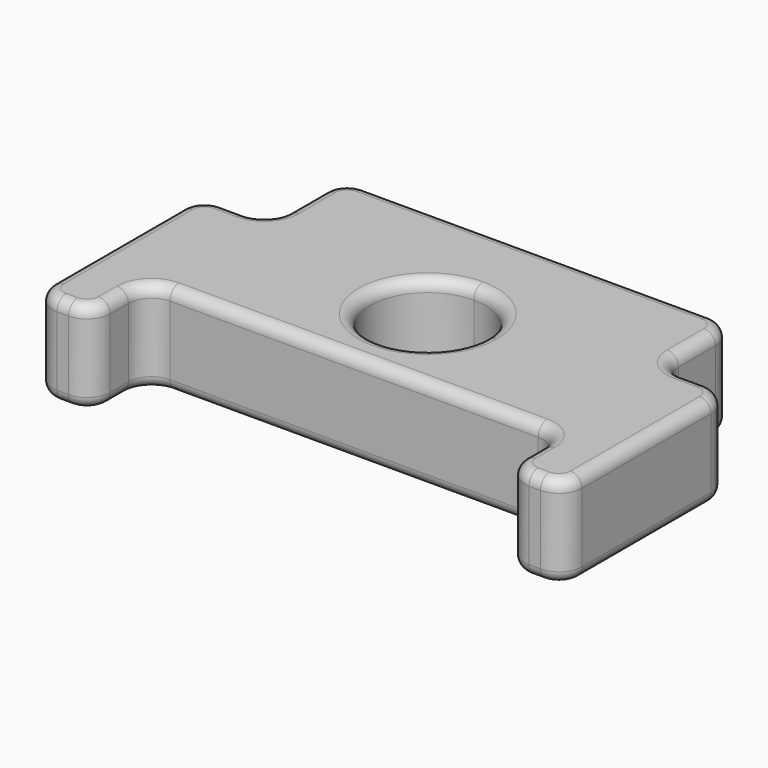
from build123d import *

# Parameters (mm, degrees)
F1_DEPTH = 4
F2_R     = 1
F3_R     = 0.5
F5_DEPTH = 4.001
F6_R     = 0.5


# Not quite as in the source:
# - a feature names something its author has since deleted; it is built from what else it names


with BuildPart() as f1:
    # F0 (on Top) → F1 (new body)
    with BuildSketch(Plane.XY):
        Polygon((9, -10), (9, -13), (11.5, -13), (11.5, -4), (8.5, -4), (8.5, 0), (-8.5, 0), (-8.5, -4), (-11.5, -4), (-11.5, -13), (-9, -13), (-9, -10), align=None)
    extrude(amount=F1_DEPTH)

    # F2
    f2_edges = [f1.edges().sort_by_distance(p)[0] for p in [
        (-9, -13, 2),
        (-9, -10, 2),
        (9, -10, 2),
        (9, -13, 2),
        (-11.5, -4, 2),
        (-8.5, -4, 2),
        (-8.5, 0, 2),
        (8.5, 0, 2),
        (8.5, -4, 2),
        (11.5, -4, 2),
        (11.5, -13, 2),
        (-11.5, -13, 2),
    ]]
    fillet(f2_edges, radius=F2_R)

    # F3
    f3_edges = [f1.edges().sort_by_distance(p)[0] for p in [
        (0, -10, 4),
        (-9, -11.5, 4),
        (9, -11.5, 4),
        (8.707107, -10.292893, 4),
        (9.292893, -12.707107, 4),
        (10.25, -13, 4),
        (-8.707107, -10.292893, 4),
        (11.207107, -12.707107, 4),
        (11.5, -8.5, 4),
        (-9.292893, -12.707107, 4),
        (11.207107, -4.292893, 4),
        (-10.25, -13, 4),
        (10, -4, 4),
        (-11.207107, -12.707107, 4),
        (8.792893, -3.707107, 4),
        (-11.5, -8.5, 4),
        (8.5, -2, 4),
        (-11.207107, -4.292893, 4),
        (8.207107, -0.292893, 4),
        (-10, -4, 4),
        (0, 0, 4),
        (-8.792893, -3.707107, 4),
        (-8.207107, -0.292893, 4),
        (-8.5, -2, 4),
        (0, -10, 0),
        (10.25, -13, 0),
        (9, -11.5, 0),
        (-9, -11.5, 0),
        (-10.25, -13, 0),
    ]]
    fillet(f3_edges, radius=F3_R)

    # F4 (on face) → F5 (cut, through all)
    with BuildSketch(Plane.XY.offset(4)):
        with BuildLine():
            ThreePointArc((2.5, -6), (1.767766953, -4.232233047), (0, -3.5))
            ThreePointArc((0, -3.5), (-1.767766953, -7.767766953), (2.5, -6))
        make_face()
    extrude(amount=-F5_DEPTH, mode=Mode.SUBTRACT)

    # F6
    f6_edges = [f1.edges().sort_by_distance(p)[0] for p in [
        (-2.5, -6, 4),
        (-2.5, -6, 0),
    ]]
    fillet(f6_edges, radius=F6_R)


solid = f1.part
